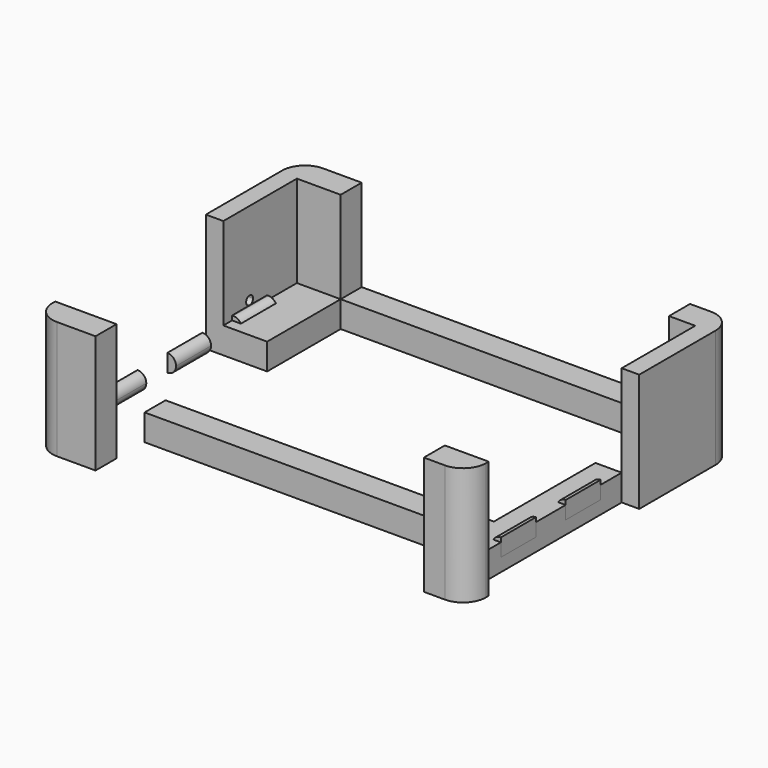
from build123d import *

# Parameters (mm, degrees)
F0_W         = 2
F0_H         = 10.5
F0_H_2       = 3
F0_W_2       = 5
F1_DEPTH     = 13.5
F0_W_3       = 3
F0_W_4       = 37.5
F2_DEPTH     = 3
F3_R         = 2.6
F3_2_R       = 2.6
F3_3_R       = 2.6
F3_4_R       = 2.6
F6_DEPTH     = 1
F7_R         = 0.99999
F7_2_R       = 0.99999
F7_3_R       = 0.99999
F10_DEPTH    = 1
F11_T1_DEPTH = 9.3301270189
F11_2_F1_R   = 0.9999
F11_2_F2_R   = 0.9999
F11_3_F1_R   = 0.9999
F11_3_F2_R   = 0.9999
F12_DEPTH    = 5
F13_DEPTH    = 5


# Not quite as in the source:
# - a fillet or chamfer that OpenCascade refuses, or shapes differently, is made with other operations: its cross-section is extruded or revolved along the edge and cut away or added
# - a fillet or chamfer is up to 0.001 mm smaller than in the source, because OpenCascade refuses the exact size
# - a feature of the source that left no trace in its solid (it failed there, or was rolled back) is left out
# - a feature names something its author has since deleted; it is built from what else it names


with BuildPart() as f1:
    # F0 (on Top) → F1 (new body)
    with BuildSketch(Plane.XY):
        with Locations((-23.75, 10.75)):
            Rectangle(F0_W, F0_H)
        with Locations((-23.75, 17.5)):
            Rectangle(F0_W, F0_H_2)
        with Locations((-20.25, 17.5)):
            Rectangle(F0_W_2, F0_H_2)
    extrude(amount=F1_DEPTH)

    # F0 (on Top) → F2 (join)
    with BuildSketch(Plane.XY):
        with Locations((1, 17.5)):
            Rectangle(F0_W_4, F0_H_2)
        with Locations((-20.25, 10.75)):
            Rectangle(F0_W_2, F0_H)
    extrude(amount=F2_DEPTH)

    # F3
    f3_edges = [f1.edges().sort_by_distance(p)[0] for p in [
        (-24.75, 19, 6.75),
    ]]
    fillet(f3_edges, radius=F3_R)

    # F9 (on face) → F10, piece 3 (join)
    with BuildSketch(Plane.YZ.offset(-22.75)):
        Polygon((6.75, 3.5), (6.75, 1.5), (9.25, 1.5), (11.75, 1.5), (11.75, 3.5), (9.25, 3.5), align=None)
    extrude(amount=F10_DEPTH)

    # F11: fillet of radius 1 on 1 edges, made by hand

    # F11_s2 → F11_t1 (cut)
    with BuildSketch(Plane.XZ.offset(-13.9150635095)):
        with BuildLine():
            ThreePointArc((-22.6160254038, 3.5), (-22.1160254038, 3.3660254038), (-21.75, 3))
            Line((-21.75, 3), (-21.75, 3.5))
            Line((-21.75, 3.5), (-22.6160254038, 3.5))
        make_face()
    extrude(amount=F11_T1_DEPTH, mode=Mode.SUBTRACT)

    # F5 (on face) → F12 (cut)
    with BuildSketch(Plane.YZ.offset(22.75)):
        with BuildLine():
            ThreePointArc((-8.75, 4), (-9.6035533906, 4.3535533906), (-9.25, 3.5))
            ThreePointArc((-9.25, 3.5), (-8.8964466094, 3.6464466094), (-8.75, 4))
        make_face()
        with BuildLine():
            ThreePointArc((-8.75, 1), (-8.8964466094, 1.3535533906), (-9.25, 1.5))
            ThreePointArc((-9.25, 1.5), (-9.6035533906, 0.6464466094), (-8.75, 1))
        make_face()
        with BuildLine():
            ThreePointArc((0.5, 4), (-0.3535533906, 4.3535533906), (0, 3.5))
            ThreePointArc((0, 3.5), (0.3535533906, 3.6464466094), (0.5, 4))
        make_face()
        with BuildLine():
            ThreePointArc((0.5, 1), (0.3535533906, 1.3535533906), (0, 1.5))
            ThreePointArc((0, 1.5), (-0.3535533906, 0.6464466094), (0.5, 1))
        make_face()
    extrude(amount=F12_DEPTH, mode=Mode.SUBTRACT)

    # F9 (on face) → F13 (cut)
    with BuildSketch(Plane.YZ.offset(-22.75)):
        with BuildLine():
            ThreePointArc((-8.75, 4), (-9.6035533906, 4.3535533906), (-9.25, 3.5))
            ThreePointArc((-9.25, 3.5), (-8.8964466094, 3.6464466094), (-8.75, 4))
        make_face()
        with BuildLine():
            ThreePointArc((0.5, 4), (-0.3535533906, 4.3535533906), (0, 3.5))
            ThreePointArc((0, 3.5), (0.3535533906, 3.6464466094), (0.5, 4))
        make_face()
        with BuildLine():
            ThreePointArc((9.75, 4), (8.8964466094, 4.3535533906), (9.25, 3.5))
            ThreePointArc((9.25, 3.5), (9.6035533906, 3.6464466094), (9.75, 4))
        make_face()
        with BuildLine():
            ThreePointArc((9.75, 1), (9.6035533906, 1.3535533906), (9.25, 1.5))
            ThreePointArc((9.25, 1.5), (8.8964466094, 0.6464466094), (9.75, 1))
        make_face()
        with BuildLine():
            ThreePointArc((0.5, 1), (0.3535533906, 1.3535533906), (0, 1.5))
            ThreePointArc((0, 1.5), (-0.3535533906, 0.6464466094), (0.5, 1))
        make_face()
        with BuildLine():
            ThreePointArc((-8.75, 1), (-8.8964466094, 1.3535533906), (-9.25, 1.5))
            ThreePointArc((-9.25, 1.5), (-9.6035533906, 0.6464466094), (-8.75, 1))
        make_face()
    extrude(amount=-F13_DEPTH, mode=Mode.SUBTRACT)


with BuildPart() as f1b:
    # F0 (on Top) → F1, piece 2 (new body)
    with BuildSketch(Plane.XY):
        with Locations((-23.75, -17.5)):
            Rectangle(F0_W, F0_H_2)
        with Locations((-20.25, -17.5)):
            Rectangle(F0_W_2, F0_H_2)
    extrude(amount=F1_DEPTH)

    # F3#2
    f3_2_edges = [f1b.edges().sort_by_distance(p)[0] for p in [
        (-24.75, -19, 6.75),
    ]]
    fillet(f3_2_edges, radius=F3_2_R)


with BuildPart() as f1c:
    # F0 (on Top) → F1, piece 3 (new body)
    with BuildSketch(Plane.XY):
        with Locations((21.25, -17.5)):
            Rectangle(F0_W_3, F0_H_2)
        with Locations((23.75, -17.5)):
            Rectangle(F0_W, F0_H_2)
    extrude(amount=F1_DEPTH)

    # F0 (on Top) → F2, piece 2 (join)
    with BuildSketch(Plane.XY):
        Polygon((22.75, 5.5), (19.75, 5.5), (19.75, -9), (19.75, -12), (19.75, -16), (22.75, -16), align=None)
        with Locations((1, -10.5)):
            Rectangle(F0_W_4, F0_H_2)
    extrude(amount=F2_DEPTH)

    # F3#3
    f3_3_edges = [f1c.edges().sort_by_distance(p)[0] for p in [
        (24.75, -19, 6.75),
    ]]
    fillet(f3_3_edges, radius=F3_3_R)


with BuildPart() as f1d:
    # F0 (on Top) → F1, piece 4 (new body)
    with BuildSketch(Plane.XY):
        with Locations((23.75, 10.75)):
            Rectangle(F0_W, F0_H)
        with Locations((23.75, 17.5)):
            Rectangle(F0_W, F0_H_2)
        with Locations((21.25, 17.5)):
            Rectangle(F0_W_3, F0_H_2)
    extrude(amount=F1_DEPTH)

    # F3#4
    f3_4_edges = [f1d.edges().sort_by_distance(p)[0] for p in [
        (24.75, 19, 6.75),
    ]]
    fillet(f3_4_edges, radius=F3_4_R)


with BuildPart() as f6:
    # F5 (on face) → F6 (new body)
    with BuildSketch(Plane.YZ.offset(22.75)):
        Polygon((-11.75, 3.5), (-11.75, 1.5), (-9.25, 1.5), (-6.75, 1.5), (-6.75, 3.5), (-9.25, 3.5), align=None)
    extrude(amount=-F6_DEPTH)

    # F7 (radius 1 in the source; OpenCascade refuses exactly that, so slightly less here)
    f7_edges = [f6.edges().sort_by_distance(p)[0] for p in [
        (21.75, -9.25, 3.5),
        (21.75, -9.25, 1.5),
    ]]
    fillet(f7_edges, radius=F7_R)


with BuildPart() as f6b:
    # F5 (on face) → F6, piece 2 (new body)
    with BuildSketch(Plane.YZ.offset(22.75)):
        Polygon((-2.5, 3.5), (-2.5, 1.5), (0, 1.5), (2.5, 1.5), (2.5, 3.5), (0, 3.5), align=None)
    extrude(amount=-F6_DEPTH)

    # F7#2 (radius 1 in the source; OpenCascade refuses exactly that, so slightly less here)
    f7_2_edges = [f6b.edges().sort_by_distance(p)[0] for p in [
        (21.75, 0, 3.5),
        (21.75, 0, 1.5),
    ]]
    fillet(f7_2_edges, radius=F7_2_R)


with BuildPart() as f6c:
    # F5 (on face) → F6, piece 3 (new body)
    with BuildSketch(Plane.YZ.offset(22.75)):
        Polygon((6.75, 3.5), (6.75, 1.5), (9.25, 1.5), (11.75, 1.5), (11.75, 3.5), (9.25, 3.5), align=None)
    extrude(amount=-F6_DEPTH)

    # F7#3 (radius 1 in the source; OpenCascade refuses exactly that, so slightly less here)
    f7_3_edges = [f6c.edges().sort_by_distance(p)[0] for p in [
        (21.75, 9.25, 1.5),
        (21.75, 9.25, 3.5),
    ]]
    fillet(f7_3_edges, radius=F7_3_R)


with BuildPart() as f10:
    # F9 (on face) → F10 (new body)
    with BuildSketch(Plane.YZ.offset(-22.75)):
        Polygon((-11.75, 3.5), (-11.75, 1.5), (-9.25, 1.5), (-6.75, 1.5), (-6.75, 3.5), (-9.25, 3.5), align=None)
    extrude(amount=F10_DEPTH)

    # F11#2: fillet of radius 1 on 2 edges, made by hand

    # F11_2_f1 (radius 1 in the source; OpenCascade refuses exactly that, so slightly less here)
    f11_2_f1_edges = [f10.edges().sort_by_distance(p)[0] for p in [
        (-21.75, -9.25, 1.5),
    ]]
    fillet(f11_2_f1_edges, radius=F11_2_F1_R)

    # F11_2_f2 (radius 1 in the source; OpenCascade refuses exactly that, so slightly less here)
    f11_2_f2_edges = [f10.edges().sort_by_distance(p)[0] for p in [
        (-21.75, -9.25, 3.5),
    ]]
    fillet(f11_2_f2_edges, radius=F11_2_F2_R)


with BuildPart() as f10b:
    # F9 (on face) → F10, piece 2 (new body)
    with BuildSketch(Plane.YZ.offset(-22.75)):
        Polygon((-2.5, 3.5), (-2.5, 1.5), (0, 1.5), (2.5, 1.5), (2.5, 3.5), (0, 3.5), align=None)
    extrude(amount=F10_DEPTH)

    # F11#3: fillet of radius 1 on 2 edges, made by hand

    # F11_3_f1 (radius 1 in the source; OpenCascade refuses exactly that, so slightly less here)
    f11_3_f1_edges = [f10b.edges().sort_by_distance(p)[0] for p in [
        (-21.75, 0, 1.5),
    ]]
    fillet(f11_3_f1_edges, radius=F11_3_F1_R)

    # F11_3_f2 (radius 1 in the source; OpenCascade refuses exactly that, so slightly less here)
    f11_3_f2_edges = [f10b.edges().sort_by_distance(p)[0] for p in [
        (-21.75, 0, 3.5),
    ]]
    fillet(f11_3_f2_edges, radius=F11_3_F2_R)


solid = Compound([f1.part, f1b.part, f1c.part, f1d.part, f6.part, f6b.part, f6c.part, f10.part, f10b.part])
